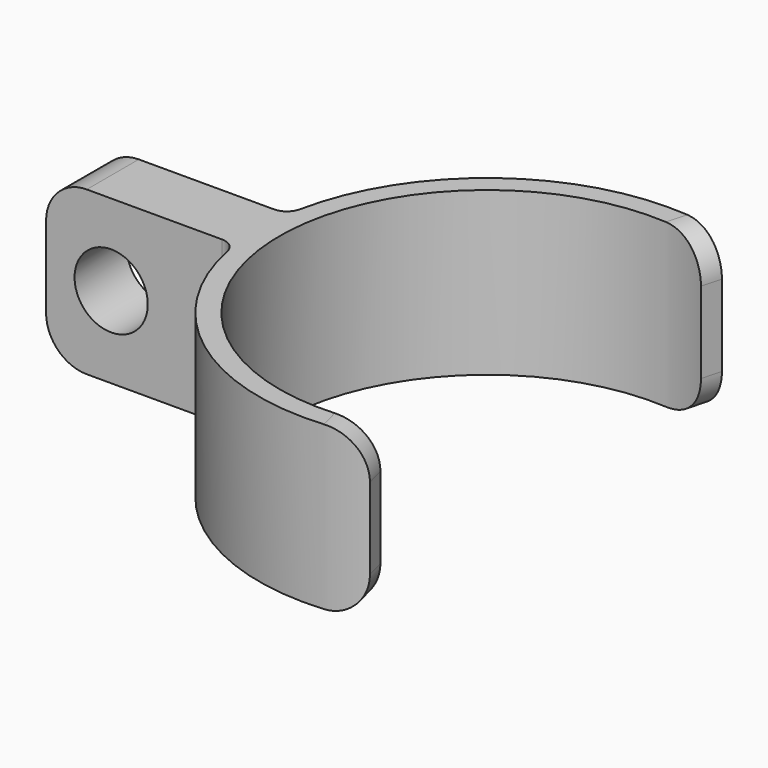
from build123d import *

# Parameters (mm, degrees)
F0_W          = 2.5
F0_H          = 20
F1_ANGLE_BACK = 105
F1_ANGLE      = 210
F2_DEPTH      = 4
F4_D          = 9
F5_R          = 2
F6_R          = 5
F7_R          = 5


# Not quite as in the source:
# - a feature names something its author has since deleted; it is built from what else it names


with BuildPart() as f1:
    # F0 (on Front) → F1 (revolve)
    with BuildSketch(Plane.XZ, mode=Mode.PRIVATE) as f1_sk:
        with Locations((16.0981313139, 0)):
            Rectangle(F0_W, F0_H)
    revolve(f1_sk.sketch.rotate(Axis((42.8481313139, 0, -3.3182863891), (0, 0, -1)), -F1_ANGLE_BACK), axis=Axis((42.8481313139, 0, -3.3182863891), (0, 0, -1)), revolution_arc=F1_ANGLE)

    # F0 (on Front) → F2 (join, symmetric)
    with BuildSketch(Plane.XZ):
        Polygon((14.8481313139, -10), (14.8481313139, 10), (-0.1518686861, 10), (-8.1518686861, 10), (-8.1518686861, -1.747650138), (-8.1518686861, -10), (-0.1518686861, -10), align=None)
        with Locations((16.0981313139, 0)):
            Rectangle(F0_W, F0_H)
    extrude(amount=F2_DEPTH, both=True)

    # F4 (through all)
    with Locations(Plane.XZ.offset(4)):
        with Locations((-0.1518686861, 0)):
            Hole(F4_D / 2)

    # F5
    f5_edges = [f1.edges().sort_by_distance(p)[0] for p in [
        (15.135318, -4, 0),
        (15.135318, 4, 0),
    ]]
    fillet(f5_edges, radius=F5_R)

    # F6
    f6_edges = [f1.edges().sort_by_distance(p)[0] for p in [
        (49.771541, -25.838516, 10),
        (49.771541, -25.838516, -10),
        (49.771541, 25.838516, -10),
        (49.771541, 25.838516, 10),
    ]]
    fillet(f6_edges, radius=F6_R)

    # F7
    f7_edges = [f1.edges().sort_by_distance(p)[0] for p in [
        (-8.151869, 0, 10),
        (-8.151869, 0, -10),
    ]]
    fillet(f7_edges, radius=F7_R)


solid = f1.part
